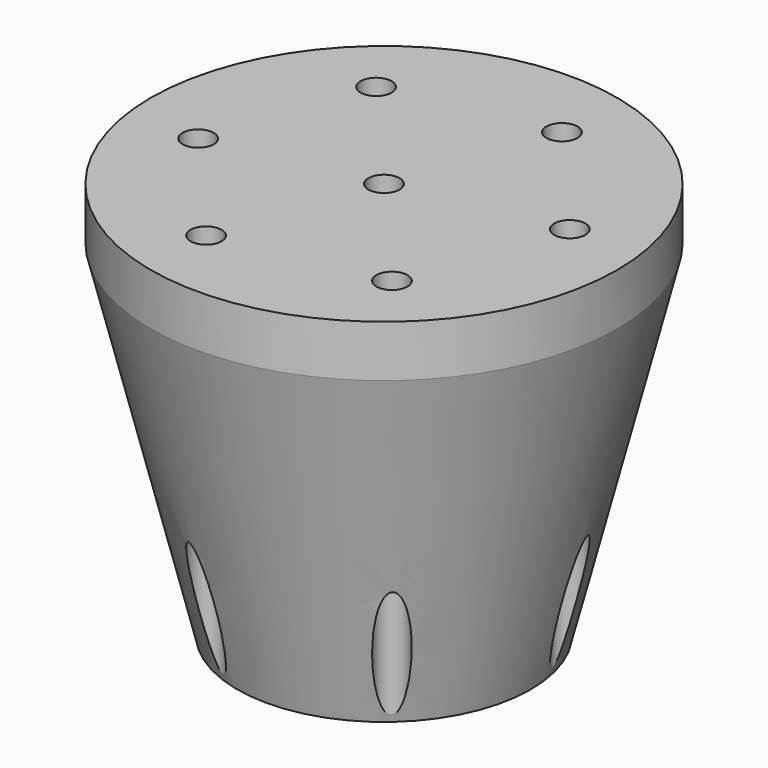
from build123d import *

# Parameters (mm, degrees)
F0_R     = 13.5
F0_R_2   = 0.9
F1_DEPTH = 23


# Not quite as in the source:
# - a fillet or chamfer that OpenCascade refuses, or shapes differently, is made with other operations: its cross-section is extruded or revolved along the edge and cut away or added


with BuildPart() as f1:
    # F0 (on Top) → F1 (new body)
    with BuildSketch(Plane.XY):
        Circle(F0_R)
        with Locations((-3.1211513103, -8.9726481319)):
            Circle(F0_R_2, mode=Mode.SUBTRACT)
        with Locations((-9.3311168766, -1.7833277421)):
            Circle(F0_R_2, mode=Mode.SUBTRACT)
        with Locations((6.2099655662, -7.1893203897)):
            Circle(F0_R_2, mode=Mode.SUBTRACT)
        with Locations((-6.2099655662, 7.1893203897)):
            Circle(F0_R_2, mode=Mode.SUBTRACT)
        Circle(F0_R_2, mode=Mode.SUBTRACT)
        with Locations((9.3311168766, 1.7833277421)):
            Circle(F0_R_2, mode=Mode.SUBTRACT)
        with Locations((3.1211513103, 8.9726481319)):
            Circle(F0_R_2, mode=Mode.SUBTRACT)
    extrude(amount=F1_DEPTH)

    # F2: chamfer of 20 x 5 on 1 edges, made by hand

    # F2_s1 → F2_t2 (revolve, cut)
    with BuildSketch(Plane.XZ):
        Polygon((13.5, 20), (8.5, 0), (13.5, 0), align=None)
    revolve(axis=Axis((0, 0, 0), (0, 0, 1)), mode=Mode.SUBTRACT)


solid = f1.part
